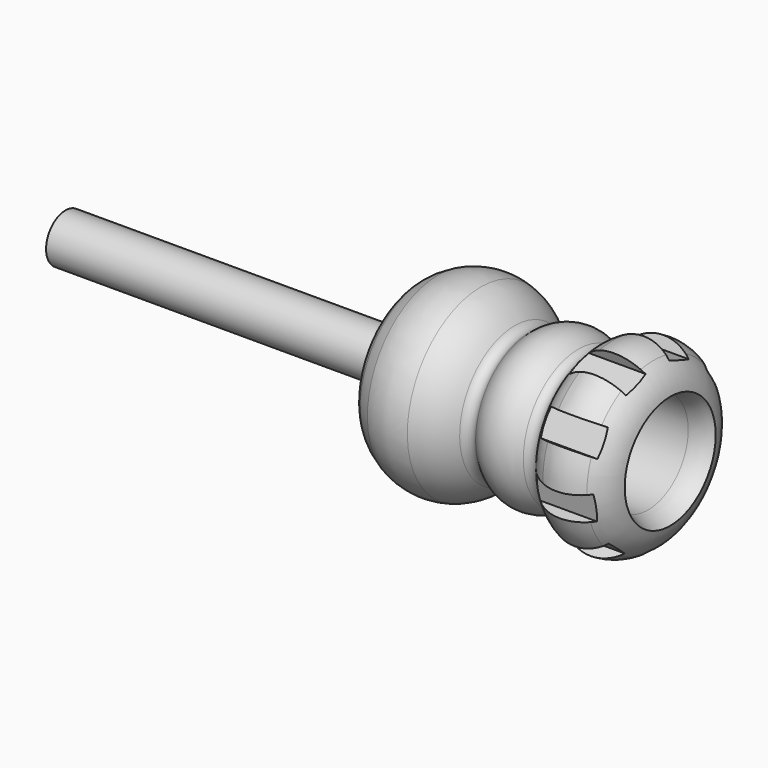
from build123d import *
from build123d import SkipClean  # not in build123d's __all__

# Parameters (mm, degrees)
F0_W          = 32.9918898642
F0_H          = 3.0656200834
F0_W_2        = 43.5025729239
F3_W          = 3.302
F3_H          = 7.62
F5_DEPTH      = 2.286
F5_DEPTH_BACK = 12.192
F4_R          = 6.35
F4_R_2        = 1.4243848289
F6_DEPTH      = 29.972
F7_DEPTH      = 90.8304


# Not quite as in the source:
# - a fillet or chamfer that OpenCascade refuses, or shapes differently, is made with other operations: its cross-section is extruded or revolved along the edge and cut away or added
# - after a boolean that leaves OpenCascade's solid faulty, fix() repairs it
# - the program builds the solid bodies; features that only make, move or delete a surface that nothing else refers to are left out


with BuildPart() as f1:
    # F0 (on Front) → F1 (revolve)
    with BuildSketch(Plane.XZ):
        with BuildLine():
            Line((-32.9918898642, 3.0656200834), (0, 3.0656200834))
            Line((0, 3.0656200834), (0, 7.1921711788))
            ThreePointArc((0, 7.1921711788), (-0.7412081671, 9.06537681), (-2.1274264505, 10.5271181533))
            ThreePointArc((-2.1274264505, 10.5271181533), (-4.5866595205, 11.4799059433), (-7.2007763421, 11.1305850192))
            ThreePointArc((-7.2007763421, 11.1305850192), (-8.6272430212, 10.27231887), (-9.7174335513, 9.0141803332))
            ThreePointArc((-9.7174335513, 9.0141803332), (-10.5964164224, 8.430696306), (-11.613028666, 8.7127672968))
            ThreePointArc((-11.613028666, 8.7127672968), (-14.7303943118, 9.8002948397), (-17.7828241898, 8.541979869))
            ThreePointArc((-17.7828241898, 8.541979869), (-18.762830138, 8.2022558028), (-19.6692659518, 8.7064365395))
            ThreePointArc((-19.6692659518, 8.7064365395), (-21.5672988363, 10.5216921139), (-23.9514680489, 11.6232450165))
            ThreePointArc((-23.9514680489, 11.6232450165), (-26.6799121824, 11.8838929117), (-29.3358409513, 11.2068500111))
            ThreePointArc((-29.3358409513, 11.2068500111), (-31.4258314596, 9.8406472706), (-32.9918898642, 7.8959027305))
            Line((-32.9918898642, 7.8959027305), (-32.9918898642, 3.0656200834))
        make_face()
        with Locations((-16.4959449321, 1.5328100417)):
            Rectangle(F0_W, F0_H)
    revolve(axis=Axis((-38.2472313941, 0, 0), (-1, 0, 0)))

    # F3 (on Right) → F5 (cut, two sides)
    with BuildSketch(Plane.YZ) as f5_sk:
        Polygon((-14.4183217137, 10.2308325115), (-16.0693217137, 7.3712166282), (-9.4702081368, 3.5612166282), (-7.8192081368, 6.4208325115), align=None)
        Polygon((-17.621327603, -1.4306461561), (-17.0479413204, -4.6824813565), (-9.5437062424, -3.3592822427), (-10.1170925251, -0.1074470423), align=None)
        Polygon((-12.5791184677, -12.4227095874), (-10.0496397165, -14.5451942746), (-5.1515981307, -8.707935618), (-7.6810768819, -6.5854509308), align=None)
        Polygon((-4.4688228527, 17.105190944), (-7.5716878865, 15.9758404307), (-4.9654943944, 8.8153826603), (-1.8626293605, 9.9447331736), align=None)
        Polygon((7.5716878865, 15.9758404307), (4.4688228527, 17.105190944), (1.8626293605, 9.9447331736), (4.9654943944, 8.8153826603), align=None)
        with Locations((0, -13.7920491397)):
            Rectangle(F3_W, F3_H)
        Polygon((10.0496397165, -14.5451942746), (12.5791184677, -12.4227095874), (7.6810768819, -6.5854509308), (5.1515981307, -8.707935618), align=None)
        Polygon((17.0479413204, -4.6824813565), (17.621327603, -1.4306461561), (10.1170925251, -0.1074470423), (9.5437062424, -3.3592822427), align=None)
        Polygon((16.0693217137, 7.3712166282), (14.4183217137, 10.2308325115), (7.8192081368, 6.4208325115), (9.4702081368, 3.5612166282), align=None)
    with SkipClean():  # cleaning this boolean's faces spoils the solid; the shape is the same uncleaned
        extrude(amount=F5_DEPTH, mode=Mode.SUBTRACT)
        extrude(f5_sk.sketch, amount=-F5_DEPTH_BACK, mode=Mode.SUBTRACT)

    # F4 (on Right) → F6 (cut)
    with BuildSketch(Plane.YZ):
        Circle(F4_R)
        Circle(F4_R_2, mode=Mode.SUBTRACT)
    extrude(amount=-F6_DEPTH, mode=Mode.SUBTRACT)

    add(f1.part.fix(), mode=Mode.REPLACE)

    # F4 (on Right) → F7 (cut)
    with BuildSketch(Plane.YZ):
        Circle(F4_R_2)
    extrude(amount=-F7_DEPTH, mode=Mode.SUBTRACT)

    # F9: fillet of radius 5.08 on 3 edges, made by hand

    # F9_s1 → F9_t2 (revolve)
    with BuildSketch(Plane.XY):
        with BuildLine():
            ThreePointArc((-29.972, 1.4243848289), (-28.4314445131, 4.9162772063), (-24.8943464745, 6.35))
            Line((-24.8943464745, 6.35), (-29.972, 6.35))
            Line((-29.972, 6.35), (-29.972, 1.4243848289))
        make_face()
    revolve(axis=Axis((-29.972, 0, 0), (1, 0, 0)))

    # F9_s3 → F9_t4 (revolve, cut)
    with BuildSketch(Plane.XY):
        with BuildLine():
            ThreePointArc((-2.8012866476, 6.35), (-1.3387153522, 6.5650965882), (0, 7.1921711788))
            Line((0, 7.1921711788), (0, 6.35))
            Line((0, 6.35), (-2.8012866476, 6.35))
        make_face()
    revolve(axis=Axis((0, 0, 0), (1, 0, 0)), mode=Mode.SUBTRACT)

    # F9_s5 → F9_t6 (revolve, cut)
    with BuildSketch(Plane.XZ):
        with BuildLine():
            ThreePointArc((-32.9918898642, 6.164993221), (-32.5057211654, 8.3336596259), (-31.1402701887, 10.0872324387))
            ThreePointArc((-31.1402701887, 10.0872324387), (-32.1652664542, 9.0753776751), (-32.9918898642, 7.8959027305))
            Line((-32.9918898642, 7.8959027305), (-32.9918898642, 6.164993221))
        make_face()
    revolve(axis=Axis((-32.9918898642, 0, 0), (-1, 0, 0)), mode=Mode.SUBTRACT)


with BuildPart() as f2:
    # F0 (on Front) → F2 (revolve)
    with BuildSketch(Plane.XZ):
        with Locations((-54.7431763262, 1.5328100417)):
            Rectangle(F0_W_2, F0_H)
    revolve(axis=Axis((-38.2472313941, 0, 0), (-1, 0, 0)))


solid = Compound([f1.part, f2.part])
